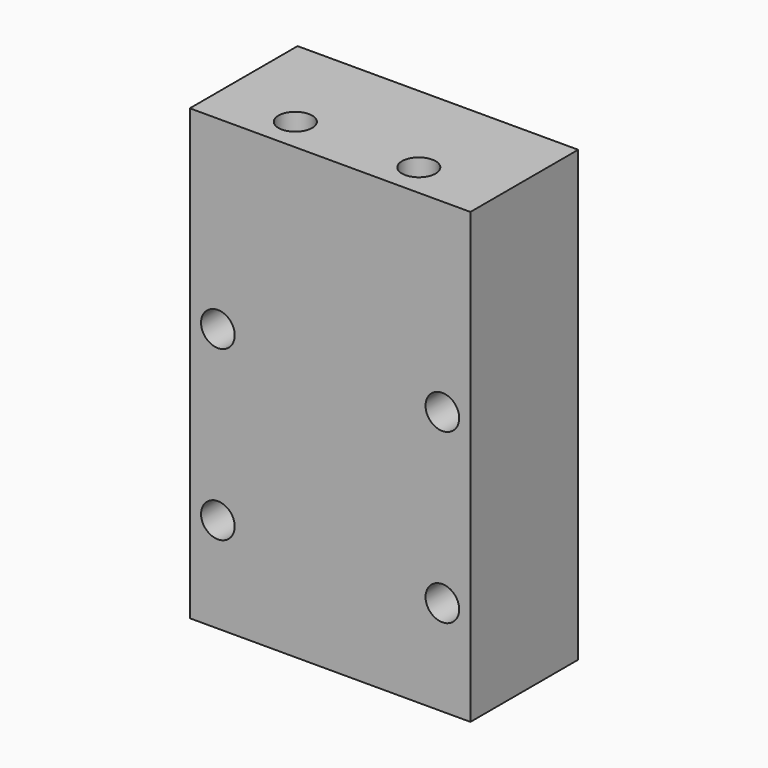
from build123d import *

# Parameters (mm, degrees)
F0_W     = 25
F0_H     = 12
F1_DEPTH = 40
F3_D     = 3
F5_D     = 3


# Not quite as in the source:
# - a feature names something its author has since deleted; it is built from what else it names


with BuildPart() as f1:
    # F0 (on Top) → F1 (new body)
    with BuildSketch(Plane.XY):
        Rectangle(F0_W, F0_H)
    extrude(amount=F1_DEPTH)

    # F3 (through all)
    with Locations(Plane.XZ.offset(6)):
        with Locations((-10, 23.5), (-10, 8.5), (10, 8.5), (10, 23.5)):
            Hole(F3_D / 2)

    # F5 (through all)
    with Locations(Plane.XY.offset(40)):
        with Locations((-5.5, -3), (5.5, -3), (-5.5, -3), (5.5, -3)):
            Hole(F5_D / 2)


solid = f1.part
